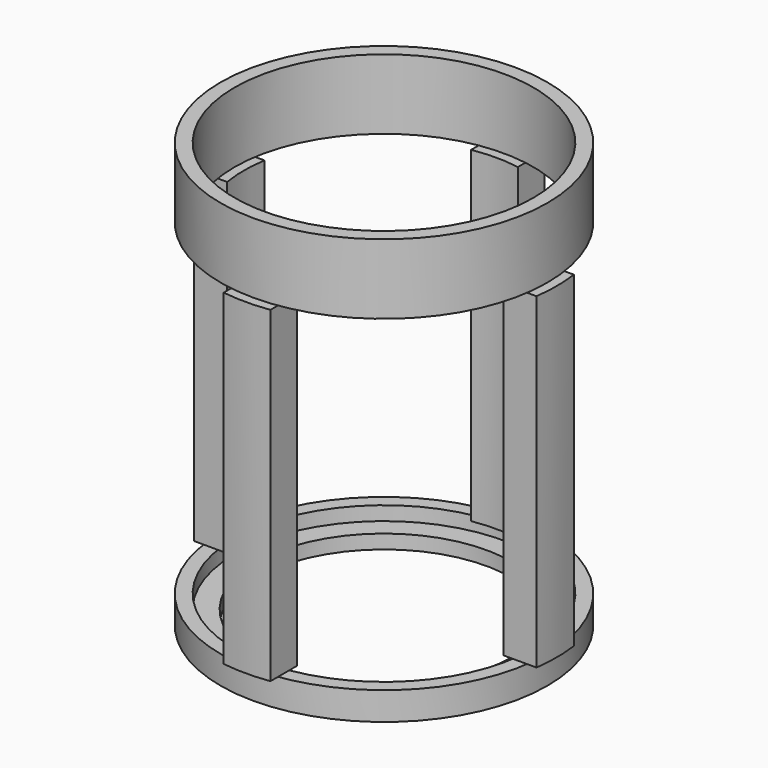
from build123d import *

# Parameters (mm, degrees)
F0_R      = 18.5
F0_R_2    = 13.75
F1_DEPTH  = 43
F2_R      = 15
F2_R_2    = 13.75
F3_DEPTH  = 41.5
F5_W      = 34.3430949748
F5_H      = 5
F5_W_2    = 5
F5_H_2    = 31.6730713844
F6_DEPTH  = 35
F7_R      = 17.5
F7_R_2    = 13.75
F8_DEPTH  = 3
F10_R     = 17.5
F10_R_2   = 16
F11_DEPTH = 7.5
F12_R     = 16
F13_DEPTH = 1.5


# Not quite as in the source:
# - a feature names something its author has since deleted; it is built from what else it names


with BuildPart() as f1:
    # F0 (on Top) → F1 (new body)
    with BuildSketch(Plane.XY):
        Circle(F0_R)
        Circle(F0_R_2, mode=Mode.SUBTRACT)
    extrude(amount=F1_DEPTH)

    # F2 (on face) → F3 (cut)
    with BuildSketch(Plane.XY.offset(43)):
        Circle(F2_R)
        Circle(F2_R_2, mode=Mode.SUBTRACT)
    extrude(amount=-F3_DEPTH, mode=Mode.SUBTRACT)

    # F5 (on offset) → F6 (intersect)
    with BuildSketch(Plane.XY.offset(3)):
        with Locations((19.6715474874, 0)):
            Rectangle(F5_W, F5_H)
        Rectangle(F5_W_2, F5_H)
        with Locations((0, 18.3365356922)):
            Rectangle(F5_W_2, F5_H_2)
        with Locations((-19.6715474874, 0)):
            Rectangle(F5_W, F5_H)
        with Locations((0, -18.3365356922)):
            Rectangle(F5_W_2, F5_H_2)
    extrude(amount=F6_DEPTH, mode=Mode.INTERSECT)


with BuildPart() as f8:
    # F7 (on Top) → F8 (new body)
    with BuildSketch(Plane.XY):
        Circle(F7_R)
        Circle(F7_R_2, mode=Mode.SUBTRACT)
    extrude(amount=F8_DEPTH)

    # F12 (on face) → F13 (cut)
    with BuildSketch(Plane.XY.offset(3)):
        Circle(F12_R)
    extrude(amount=-F13_DEPTH, mode=Mode.SUBTRACT)


with BuildPart() as f11:
    # F10 (on offset) → F11 (new body)
    with BuildSketch(Plane.XY.offset(38)):
        Circle(F10_R)
        Circle(F10_R_2, mode=Mode.SUBTRACT)
    extrude(amount=F11_DEPTH)


solid = Compound([f1.part, f8.part, f11.part])
